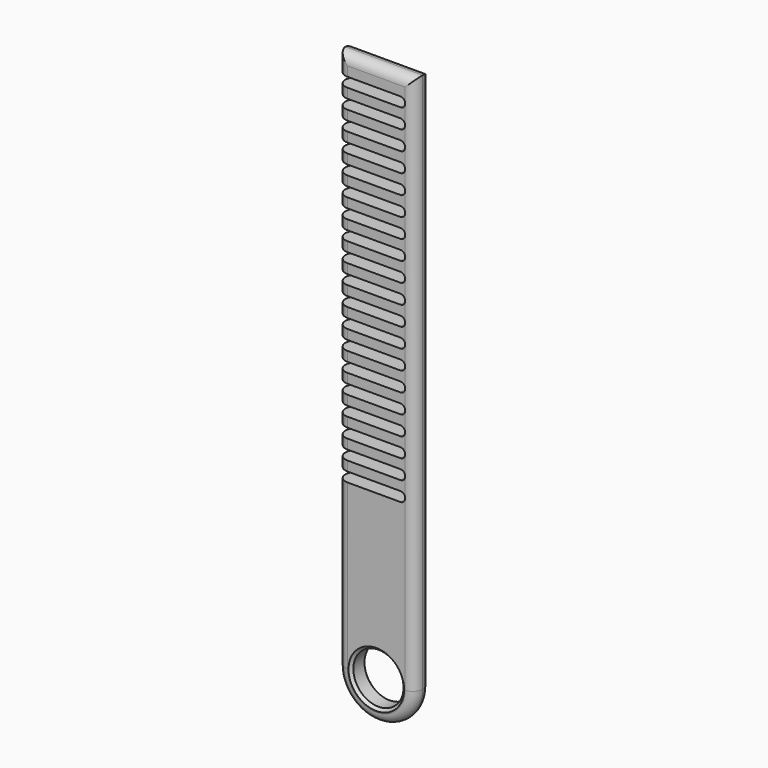
from build123d import *

# Parameters (mm, degrees)
F0_R     = 12.7
F0_R_2   = 8.255
F1_DEPTH = 3.175
F3_DEPTH = 3.175
F4_R     = 3.17499
F5_SIZE  = 0.889
F6_W     = 19.05001
F6_H     = 3.175
F6_W_2   = 3.2763721661
F7_DEPTH = 25.4
F8_R     = 1.58749


# Not quite as in the source:
# - a fillet or chamfer is up to 0.001 mm smaller than in the source, because OpenCascade refuses the exact size
# - ends of sketch curves that miss each other by under 0.0002 mm in the source are joined


with BuildPart() as f1:
    # F0 (on Front) → F1 (new body, symmetric)
    with BuildSketch(Plane.XZ):
        with Locations((0, -63.5)):
            Circle(F0_R)
        with Locations((0, -63.5)):
            Circle(F0_R_2, mode=Mode.SUBTRACT)
    extrude(amount=F1_DEPTH, both=True)

    # F2 (on Front) → F3 (join, symmetric)
    with BuildSketch(Plane.XZ):
        with BuildLine():
            Line((12.7, 114.2999971132), (-12.7, 114.2999971132))
            Line((-12.7, 114.2999971132), (-12.7, -63.5000028868))
            ThreePointArc((-12.7, -63.5000028868), (-1.4434e-06, -50.8), (12.7, -63.5))
            Line((12.7, -63.5), (12.7, 114.2999971132))
        make_face()
    extrude(amount=F3_DEPTH, both=True)

    # F4 (radius 3.175 in the source; OpenCascade refuses exactly that, so slightly less here)
    f4_edges = [f1.edges().sort_by_distance(p)[0] for p in [
        (12.7, -3.175, 25.399999),
        (12.7, 3.175, 25.399999),
        (0, -3.175, 114.299997),
        (0, 3.175, 114.299997),
    ]]
    fillet(f4_edges, radius=F4_R)

    # F5
    f5_edges = [f1.edges().sort_by_distance(p)[0] for p in [
        (-8.255, -3.175, -63.5),
        (-8.255, 3.175, -63.5),
    ]]
    chamfer(f5_edges, length=F5_SIZE)

    # F6 (on face) → F7 (cut)
    with BuildSketch(Plane.XZ.offset(3.175)):
        with Locations((-5e-06, 106.3624971132)):
            Rectangle(F6_W, F6_H)
        with Locations((-5e-06, 100.0124971132)):
            Rectangle(F6_W, F6_H)
        with Locations((-5e-06, 93.6624971132)):
            Rectangle(F6_W, F6_H)
        with Locations((-5e-06, 87.3124971132)):
            Rectangle(F6_W, F6_H)
        with Locations((-5e-06, 80.9624971132)):
            Rectangle(F6_W, F6_H)
        with Locations((-5e-06, 74.6124971132)):
            Rectangle(F6_W, F6_H)
        with Locations((-5e-06, 68.2624971132)):
            Rectangle(F6_W, F6_H)
        with Locations((-5e-06, 61.9124971132)):
            Rectangle(F6_W, F6_H)
        with Locations((-5e-06, 55.5624971132)):
            Rectangle(F6_W, F6_H)
        with Locations((-5e-06, 49.2124971132)):
            Rectangle(F6_W, F6_H)
        with Locations((-5e-06, 42.8624971132)):
            Rectangle(F6_W, F6_H)
        with Locations((-5e-06, 36.5124971132)):
            Rectangle(F6_W, F6_H)
        with Locations((-5e-06, 30.1624971132)):
            Rectangle(F6_W, F6_H)
        with Locations((-5e-06, 23.8124971132)):
            Rectangle(F6_W, F6_H)
        with Locations((-5e-06, 17.4624971132)):
            Rectangle(F6_W, F6_H)
        with Locations((-5e-06, 11.1124971132)):
            Rectangle(F6_W, F6_H)
        with Locations((-5e-06, 4.7624971132)):
            Rectangle(F6_W, F6_H)
        with Locations((-5e-06, -1.5875028868)):
            Rectangle(F6_W, F6_H)
        with Locations((-5e-06, -7.9375028868)):
            Rectangle(F6_W, F6_H)
        with Locations((-11.1631960831, 106.3624971132)):
            Rectangle(F6_W_2, F6_H)
        with Locations((-11.1631960831, 100.0124971132)):
            Rectangle(F6_W_2, F6_H)
        with Locations((-11.1631960831, 93.6624971132)):
            Rectangle(F6_W_2, F6_H)
        with Locations((-11.1631960831, 87.3124971132)):
            Rectangle(F6_W_2, F6_H)
        with Locations((-11.1631960831, 80.9624971132)):
            Rectangle(F6_W_2, F6_H)
        with Locations((-11.1631960831, 74.6124971132)):
            Rectangle(F6_W_2, F6_H)
        with Locations((-11.1631960831, -7.9375028868)):
            Rectangle(F6_W_2, F6_H)
        with Locations((-11.1631960831, -1.5875028868)):
            Rectangle(F6_W_2, F6_H)
        with Locations((-11.1631960831, 4.7624971132)):
            Rectangle(F6_W_2, F6_H)
        with Locations((-11.1631960831, 11.1124971132)):
            Rectangle(F6_W_2, F6_H)
        with Locations((-11.1631960831, 17.4624971132)):
            Rectangle(F6_W_2, F6_H)
        with Locations((-11.1631960831, 23.8124971132)):
            Rectangle(F6_W_2, F6_H)
        with Locations((-11.1631960831, 30.1624971132)):
            Rectangle(F6_W_2, F6_H)
        with Locations((-11.1631960831, 36.5124971132)):
            Rectangle(F6_W_2, F6_H)
        with Locations((-11.1631960831, 42.8624971132)):
            Rectangle(F6_W_2, F6_H)
        with Locations((-11.1631960831, 49.2124971132)):
            Rectangle(F6_W_2, F6_H)
        with Locations((-11.1631960831, 55.5624971132)):
            Rectangle(F6_W_2, F6_H)
        with Locations((-11.1631960831, 61.9124971132)):
            Rectangle(F6_W_2, F6_H)
        with Locations((-11.1631960831, 68.2624971132)):
            Rectangle(F6_W_2, F6_H)
    extrude(amount=-F7_DEPTH, mode=Mode.SUBTRACT)

    # F8 (radius 1.5875 in the source; OpenCascade refuses exactly that, so slightly less here)
    f8_edges = [f1.edges().sort_by_distance(p)[0] for p in [
        (9.525, 0, 107.949997),
        (9.525, 0, 104.774997),
        (9.525, 0, 101.599997),
        (9.525, 0, 98.424997),
        (9.525, 0, 92.074997),
        (9.525, 0, 85.724997),
        (9.525, 0, 79.374997),
        (9.525, 0, 73.024997),
        (9.525, 0, 66.674997),
        (9.525, 0, 60.324997),
        (9.525, 0, 53.974997),
        (9.525, 0, 47.624997),
        (9.525, 0, 41.274997),
        (9.525, 0, 34.924997),
        (9.525, 0, 28.574997),
        (9.525, 0, 22.224997),
        (9.525, 0, 15.874997),
        (9.525, 0, 9.524997),
        (9.525, 0, 3.174997),
        (9.525, 0, -3.175003),
        (9.525, 0, -9.525003),
        (9.525, 0, -6.350003),
        (9.525, 0, -3e-06),
        (9.525, 0, 6.349997),
        (9.525, 0, 12.699997),
        (9.525, 0, 19.049997),
        (9.525, 0, 25.399997),
        (9.525, 0, 31.749997),
        (9.525, 0, 38.099997),
        (9.525, 0, 44.449997),
        (9.525, 0, 50.799997),
        (9.525, 0, 57.149997),
        (9.525, 0, 63.499997),
        (9.525, 0, 69.849997),
        (9.525, 0, 76.199997),
        (9.525, 0, 82.549997),
        (9.525, 0, 88.899997),
        (9.525, 0, 95.249997),
    ]]
    fillet(f8_edges, radius=F8_R)


solid = f1.part
